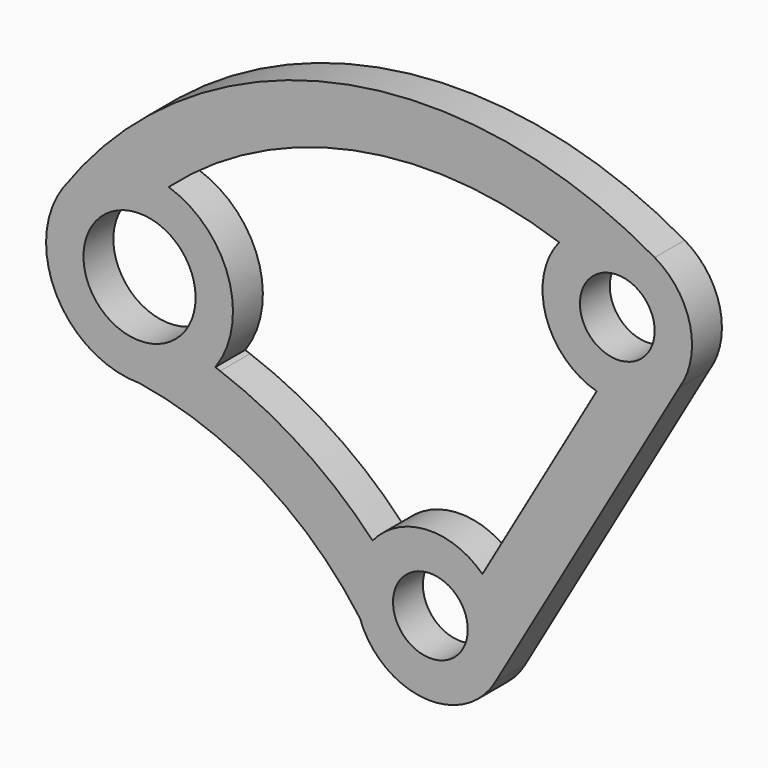
from build123d import *

# Parameters (mm, degrees)
F0_R     = 15
F0_R_2   = 10
F1_DEPTH = 10


# Not quite as in the source:
# - ends of sketch curves that miss each other by under 0.0002 mm in the source are joined


with BuildPart() as f1:
    # F0 (on Front) → F1 (new body)
    with BuildSketch(Plane.XZ):
        with BuildLine():
            ThreePointArc((-77.8194442075, 29.4897614533), (-44.7134784315, 17.2871063454), (-18.8426622217, -6.704780414))
            ThreePointArc((-18.8426622217, -6.704780414), (-1.8148984382, -19.9174833666), (17.3205080757, -10))
            Line((17.3205080757, -10), (17.2196907343, -9.9417930808))
            Line((17.2196907343, -9.9417930808), (18.301055835, -8.0666818038))
            Line((18.301055835, -8.0666818038), (65.8985825054, 74.4684942965))
            ThreePointArc((65.8985825054, 74.4684942965), (66.2472754238, 74.9395201306), (66.5820179406, 75.4205601863))
            ThreePointArc((66.5820179406, 75.4205601863), (69.4871465026, 91.102664953), (60, 103.9230484541))
            ThreePointArc((60, 103.9230484541), (-25.9727536726, 117.1555208544), (-98.2982453147, 68.8291723621))
            ThreePointArc((-98.2982453147, 68.8291723621), (-99.9947150369, 42.9460461225), (-77.8194442075, 29.4897614533))
        make_face()
        with BuildLine():
            ThreePointArc((8.590003141, 5.1197505835), (9.6410588477, 2.655180652), (10, 0))
            ThreePointArc((10, 0), (-9.6410588477, -2.655180652), (8.590003141, 5.1197505835))
        make_face(mode=Mode.SUBTRACT)
        with Locations((-77.8194442075, 54.4897614533)):
            Circle(F0_R, mode=Mode.SUBTRACT)
        with BuildLine():
            Line((44.4926580322, 67.3757573805), (13.9195380637, 14.3612833721))
            ThreePointArc((13.9195380637, 14.3612833721), (-1.1386278406, 19.9675618602), (-15.461870052, 12.6858414973))
            ThreePointArc((-15.461870052, 12.6858414973), (-34.2806761155, 28.431524103), (-56.2400022895, 39.3796735521))
            ThreePointArc((-56.2400022895, 39.3796735521), (-56.8984637414, 39.6141223401), (-57.5584712538, 39.84418277))
            ThreePointArc((-57.5584712538, 39.84418277), (-57.4489819567, 39.9968574072), (-57.3406431002, 40.1503505446))
            ThreePointArc((-57.3406431002, 40.1503505446), (-54.0993659231, 62.3864624217), (-70.0220352349, 78.2426647141))
            ThreePointArc((-70.0220352349, 78.2426647141), (-20.6376982657, 102.9518596738), (34.4547303835, 99.1860451586))
            ThreePointArc((34.4547303835, 99.1860451586), (30.9270685064, 80.5839621211), (44.4926580322, 67.3757573805))
        make_face(mode=Mode.SUBTRACT)
        with Locations((50, 86.6025403784)):
            Circle(F0_R_2, mode=Mode.SUBTRACT)
        with BuildLine():
            Line((17.2196907343, -9.9417930808), (17.3205080757, -10))
            ThreePointArc((17.3205080757, -10), (17.836994805, -9.0466356358), (18.301055835, -8.0666818038))
            Line((18.301055835, -8.0666818038), (17.2196907343, -9.9417930808))
        make_face()
        with BuildLine():
            ThreePointArc((18.301055835, -8.0666818038), (17.836994805, -9.0466356358), (17.3205080757, -10))
            Line((17.3205080757, -10), (66.5820179406, 75.4205601863))
            ThreePointArc((66.5820179406, 75.4205601863), (66.2472754238, 74.9395201306), (65.8985825054, 74.4684942965))
            Line((65.8985825054, 74.4684942965), (18.301055835, -8.0666818038))
        make_face()
    extrude(amount=F1_DEPTH)


solid = f1.part
